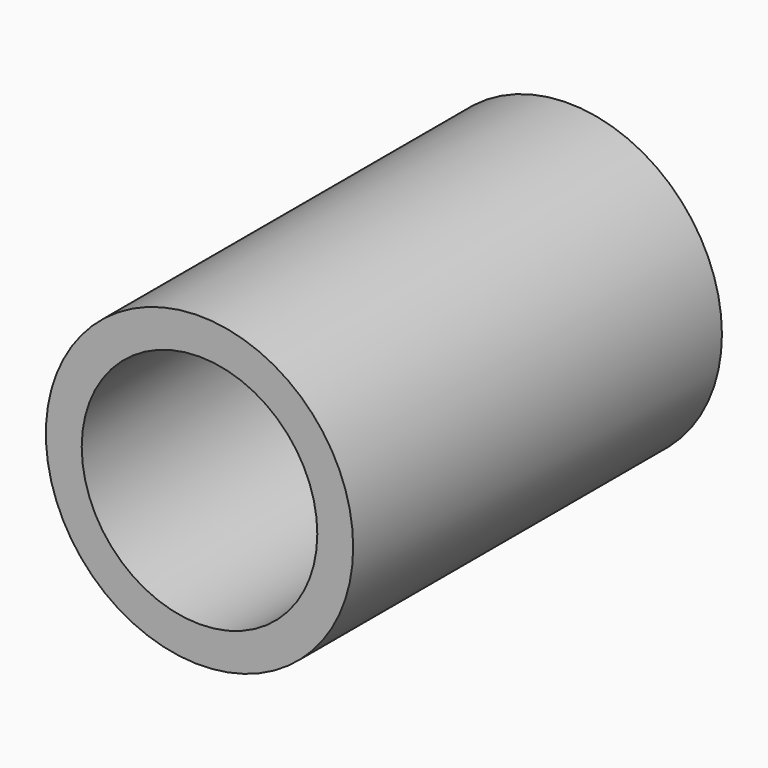
from build123d import *

# Parameters (mm, degrees)
F3_R     = 7.5
F3_R_2   = 4
F4_DEPTH = 22.5
F5_R     = 5.75
F5_R_2   = 4
F6_DEPTH = 20


# Not quite as in the source:
# - the program builds the solid bodies; features that only make, move or delete a surface that nothing else refers to are left out


with BuildPart() as f4:
    # F3 (on Front) → F4 (new body)
    with BuildSketch(Plane.XZ):
        Circle(F3_R)
        Circle(F3_R_2, mode=Mode.SUBTRACT)
    extrude(amount=-F4_DEPTH)

    # F5 (on face) → F6 (cut)
    with BuildSketch(Plane.XZ):
        Circle(F5_R)
        Circle(F5_R_2, mode=Mode.SUBTRACT)
    extrude(amount=-F6_DEPTH, mode=Mode.SUBTRACT)


solid = f4.part
